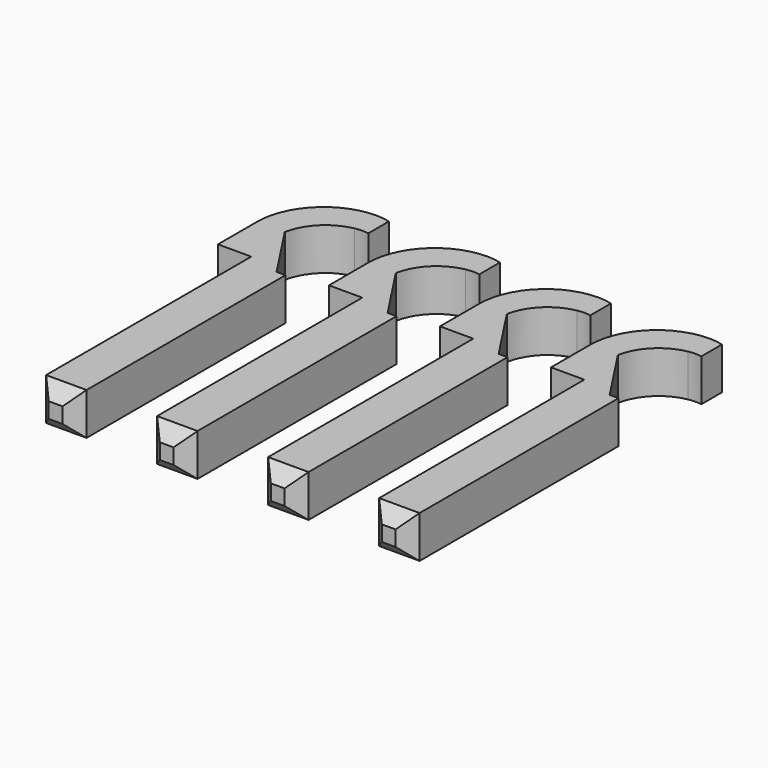
from build123d import *

# Parameters (mm, degrees)
F1_DEPTH = 4.826
F2_SIZE  = 1.524
F3_SIZE  = 1.524


# Not quite as in the source:
# - a feature names something its author has since deleted; it is built from what else it names


with BuildPart() as f1:
    # F0 (on Top) → F1 (new body)
    with BuildSketch(Plane.XY):
        with BuildLine():
            Line((3.1470672374, 30.861), (3.1470672374, 0))
            Line((3.1470672374, 0), (7.7749327626, 0))
            Line((7.7749327626, 0), (7.7749327626, 29.972))
            Line((7.7749327626, 29.972), (6.7589327626, 29.972))
            Line((6.7589327626, 29.972), (2.5120672374, 36.449))
            ThreePointArc((2.5120672374, 36.449), (4.0518978925, 39.3541693448), (6.9570672374, 40.894))
            ThreePointArc((6.9570672374, 40.894), (7.724416919, 40.973720593), (8.4941043234, 40.921163897))
            Line((8.4941043234, 40.921163897), (8.4941043234, 43.8536204909))
            ThreePointArc((8.4941043234, 43.8536204909), (7.7310836788, 44.0005455178), (6.9570672374, 44.069))
            ThreePointArc((6.9570672374, 44.069), (1.5689135647, 41.8371536726), (-0.6629327626, 36.449))
            Line((-0.6629327626, 36.449), (-0.6629327626, 30.861))
            Line((-0.6629327626, 30.861), (3.1470672374, 30.861))
        make_face()
    extrude(amount=F1_DEPTH)

    # F2
    f2_edges = [f1.edges().sort_by_distance(p)[0] for p in [
        (5.461, 0, 0),
        (3.147067, 0, 2.413),
        (5.461, 0, 4.826),
    ]]
    chamfer(f2_edges, length=F2_SIZE)

    # F3
    f3_edges = [f1.edges().sort_by_distance(p)[0] for p in [
        (7.774933, 0, 2.413),
    ]]
    chamfer(f3_edges, length=F3_SIZE)


with BuildPart() as f4_1:
    # F4: copy of F1
    add(f1.part.moved(Location((12.7, 0, 0))))


with BuildPart() as f5_1:
    # F5: copy of F4_1
    add(f4_1.part.moved(Location((12.7, 0, 0))))


with BuildPart() as f6_1:
    # F6: copy of F5_1
    add(f5_1.part.moved(Location((12.7, 0, 0))))


solid = Compound([f1.part, f4_1.part, f5_1.part, f6_1.part])
